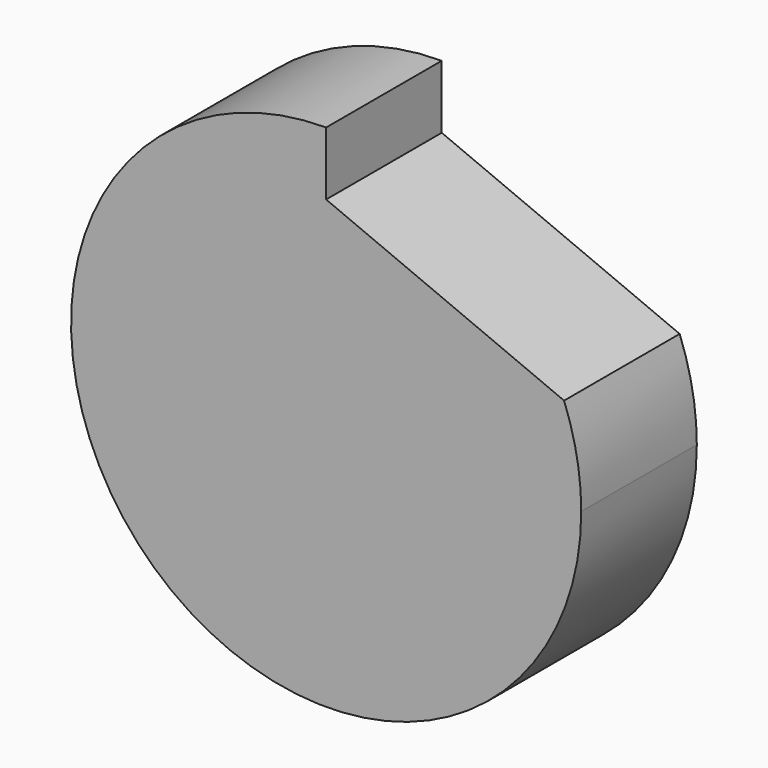
from build123d import *

# Parameters (mm, degrees)
F1_DEPTH = 25.4


# Not quite as in the source:
# - the program builds the solid bodies; features that only make, move or delete a surface that nothing else refers to are left out


with BuildPart() as f1:
    # F0 (on Front) → F1 (new body)
    with BuildSketch(Plane.XZ):
        with BuildLine():
            ThreePointArc((0, 44.8469221637), (-44.8469221637, 0), (0, -44.8469221637))
            Line((0, -44.8469221637), (0, 33.7025374174))
            Line((0, 33.7025374174), (0, 44.8469221637))
        make_face()
        with BuildLine():
            ThreePointArc((0, -44.8469221637), (31.7115627773, -31.7115627773), (44.8469221637, 0))
            ThreePointArc((44.8469221637, 0), (44.0857340296, 8.2276656851), (41.8280089648, 16.176034545))
            Line((41.8280089648, 16.176034545), (0, 33.7025374174))
            Line((0, 33.7025374174), (0, -44.8469221637))
        make_face()
    extrude(amount=F1_DEPTH)


solid = f1.part
